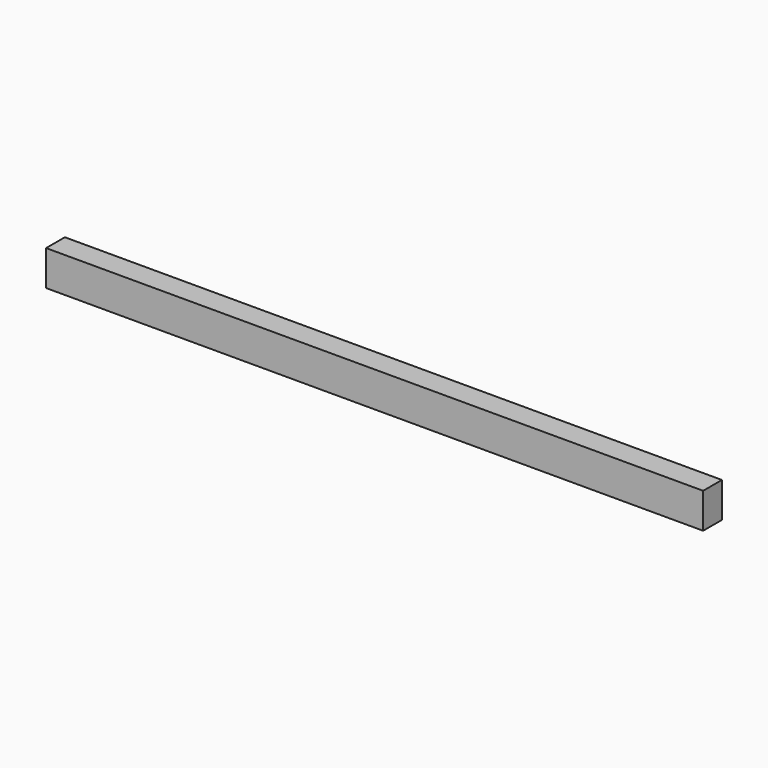
from build123d import *

# Parameters (mm, degrees)
F0_W     = 355.6
F0_H     = 19.05
F1_DEPTH = 12.7


# Not quite as in the source:
# - a feature names something its author has since deleted; it is built from what else it names


with BuildPart() as f1:
    # F0 (on Front) → F1 (new body)
    with BuildSketch(Plane.XZ):
        with Locations((116.8400510788, 144.9867119074)):
            Rectangle(F0_W, F0_H)
    extrude(amount=F1_DEPTH)


solid = f1.part
